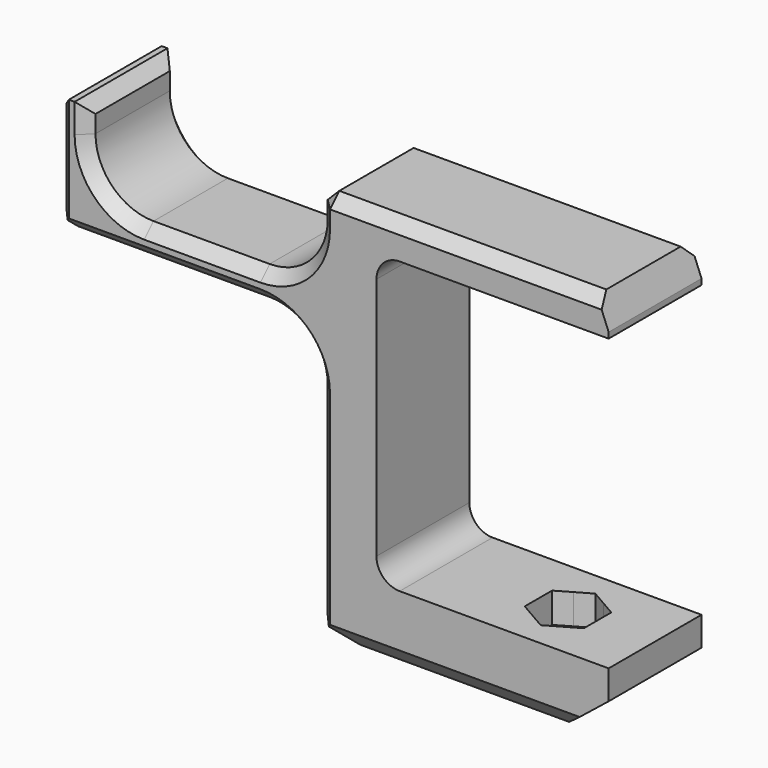
from build123d import *

# Parameters (mm, degrees)
F0_W       = 50.8
F0_H       = 6.35
F0_H_2     = 7.62
F0_H_3     = 16.51
F1_DEPTH   = 25.4
F2_R       = 12.7
F3_SIZE    = 2.54
F4_R       = 12.7
F5_SIZE    = 2.54
F6_R       = 5.08
F8_C1_SIZE = 5.08
F8_C2_SIZE = 5.08
F8_C3_SIZE = 5.08
F9_SIZE2   = 12.7
F9_SIZE    = 10.16
F10_SIZE2  = 6.35
F10_SIZE   = 2.54
F11_DEPTH  = 6.604
F12_START  = -9.906
F12_DEPTH  = 6.605
F13_D      = 8.128
F13_DEPTH  = 16.511


with BuildPart() as f1:
    # F0 (on Front) → F1 (new body)
    with BuildSketch(Plane.XZ):
        Polygon((-63.5, 19.1297054841), (-63.5, 25.4797054841), (-63.5, 44.5297054841), (-69.85, 44.5297054841), (-69.85, 19.1297054841), align=None)
        with Locations((-38.1, 22.3047054841)):
            Rectangle(F0_W, F0_H)
        Polygon((0, 36.9097054841), (0, 44.5297054841), (-12.7, 44.5297054841), (-12.7, 25.4797054841), (-12.7, 19.1297054841), (-12.7, -43.1002945159), (0, -43.1002945159), (0, -26.5902945159), align=None)
        with Locations((25.4, 40.7197054841)):
            Rectangle(F0_W, F0_H_2)
        with Locations((25.4, -34.8452945159)):
            Rectangle(F0_W, F0_H_3)
    extrude(amount=F1_DEPTH)

    # F2
    f2_edges = [f1.edges().sort_by_distance(p)[0] for p in [
        (-12.7, -12.7, 25.479705),
        (-63.5, -12.7, 25.479705),
    ]]
    fillet(f2_edges, radius=F2_R)

    # F3
    f3_edges = [f1.edges().sort_by_distance(p)[0] for p in [
        (-63.5, -12.7, 44.529705),
        (-69.85, 0, 31.829705),
        (-69.85, -12.7, 44.529705),
        (-69.85, -25.4, 31.829705),
        (-59.780256, -25.4, 29.199449),
        (-38.1, 0, 25.479705),
        (-12.7, -12.7, 44.529705),
        (19.05, -25.4, 44.529705),
        (19.05, 0, 44.529705),
        (-69.85, -12.7, 19.129705),
    ]]
    chamfer(f3_edges, length=F3_SIZE)

    # F4
    f4_edges = [f1.edges().sort_by_distance(p)[0] for p in [
        (-12.7, -12.7, 19.129705),
    ]]
    fillet(f4_edges, radius=F4_R)

    # F5
    f5_edges = [f1.edges().sort_by_distance(p)[0] for p in [
        (-12.7, -25.4, -18.335295),
        (-12.7, 0, -18.335295),
    ]]
    chamfer(f5_edges, length=F5_SIZE)

    # F6
    f6_edges = [f1.edges().sort_by_distance(p)[0] for p in [
        (0, -12.7, 36.909705),
        (0, -12.7, -26.590295),
    ]]
    fillet(f6_edges, radius=F6_R)

    # F8: chamfer of 5.08 on 5 edges, made by hand

    # F8_c1
    f8_c1_edges = [f1.edges().sort_by_distance(p)[0] for p in [
        (20.32, 0, -43.1002945159),
    ]]
    chamfer(f8_c1_edges, length=F8_C1_SIZE)

    # F8_c2
    f8_c2_edges = [f1.edges().sort_by_distance(p)[0] for p in [
        (-12.7, -13.97, -43.1002945159),
    ]]
    chamfer(f8_c2_edges, length=F8_C2_SIZE)

    # F8_c3
    f8_c3_edges = [f1.edges().sort_by_distance(p)[0] for p in [
        (21.59, -25.4, -43.1002945159),
    ]]
    chamfer(f8_c3_edges, length=F8_C3_SIZE)

    # F9
    f9_edges = [f1.edges().sort_by_distance(p)[0] for p in [
        (50.8, -12.7, -43.100295),
    ]]
    f9_side = f1.faces().sort_by_distance((50.8, -12.7, -34.415021))[0]
    chamfer(f9_edges, length=F9_SIZE, length2=F9_SIZE2, reference=f9_side)

    # F10
    f10_edges = [f1.edges().sort_by_distance(p)[0] for p in [
        (50.8, -12.7, 44.529705),
    ]]
    f10_side = f1.faces().sort_by_distance((20.32, -12.7, 44.529705))[0]
    chamfer(f10_edges, length=F10_SIZE, length2=F10_SIZE2, reference=f10_side)

    # F7 (on face) → F11 (cut)
    with BuildSketch(Plane.XY.offset(-26.5902945159)):
        with BuildLine():
            Line((25.273, -16.4394976935), (28.5114998927, -18.3092464784))
            ThreePointArc((28.5114998927, -18.3092464784), (26.1407534287, -15.9384999464), (25.273, -12.7))
            Line((25.273, -12.7), (25.273, -16.4394976935))
        make_face()
        with BuildLine():
            ThreePointArc((25.273, -12.7), (26.1407534711, -9.4614999803), (28.5115000394, -7.0907534369))
            Line((28.5115000394, -7.0907534369), (25.273, -8.9605023065))
            Line((25.273, -8.9605023065), (25.273, -12.7))
        make_face()
        with BuildLine():
            ThreePointArc((28.5115000394, -7.0907534369), (31.7500001819, -6.223), (34.9885002756, -7.0907536188))
            Line((34.9885002756, -7.0907536188), (31.75, -5.2210046129))
            Line((31.75, -5.2210046129), (28.5115000394, -7.0907534369))
        make_face()
        with BuildLine():
            ThreePointArc((34.9885002756, -7.0907536188), (37.3592466199, -9.4615001378), (38.227, -12.7))
            Line((38.227, -12.7), (38.227, -8.9605023065))
            Line((38.227, -8.9605023065), (34.9885002756, -7.0907536188))
        make_face()
        with BuildLine():
            Line((38.227, -16.4394976935), (38.227, -12.7))
            ThreePointArc((38.227, -12.7), (37.3592466025, -15.9384998923), (34.9885002155, -18.3092464159))
            Line((34.9885002155, -18.3092464159), (38.227, -16.4394976935))
        make_face()
        with BuildLine():
            Line((31.75, -20.1789953871), (34.9885002155, -18.3092464159))
            ThreePointArc((34.9885002155, -18.3092464159), (31.7500000625, -19.177), (28.5114998927, -18.3092464784))
            Line((28.5114998927, -18.3092464784), (31.75, -20.1789953871))
        make_face()
        with BuildLine():
            ThreePointArc((34.9885002155, -18.3092464159), (37.3592466025, -15.9384998923), (38.227, -12.7))
            ThreePointArc((38.227, -12.7), (37.3592466199, -9.4615001378), (34.9885002756, -7.0907536188))
            ThreePointArc((34.9885002756, -7.0907536188), (31.7500001819, -6.223), (28.5115000394, -7.0907534369))
            ThreePointArc((28.5115000394, -7.0907534369), (26.1407534711, -9.4614999803), (25.273, -12.7))
            ThreePointArc((25.273, -12.7), (26.1407534287, -15.9384999464), (28.5114998927, -18.3092464784))
            ThreePointArc((28.5114998927, -18.3092464784), (31.7500000625, -19.177), (34.9885002155, -18.3092464159))
        make_face()
    extrude(amount=-F11_DEPTH, mode=Mode.SUBTRACT)

    # F7 (on face) → F12 (cut)
    with BuildSketch(Plane.XY.offset(-26.5902945159).offset(F12_START)):
        with BuildLine():
            ThreePointArc((34.9885002155, -18.3092464159), (37.3592466025, -15.9384998923), (38.227, -12.7))
            ThreePointArc((38.227, -12.7), (37.3592466199, -9.4615001378), (34.9885002756, -7.0907536188))
            ThreePointArc((34.9885002756, -7.0907536188), (31.7500001819, -6.223), (28.5115000394, -7.0907534369))
            ThreePointArc((28.5115000394, -7.0907534369), (26.1407534711, -9.4614999803), (25.273, -12.7))
            ThreePointArc((25.273, -12.7), (26.1407534287, -15.9384999464), (28.5114998927, -18.3092464784))
            ThreePointArc((28.5114998927, -18.3092464784), (31.7500000625, -19.177), (34.9885002155, -18.3092464159))
        make_face()
        with BuildLine():
            Line((38.227, -16.4394976935), (38.227, -12.7))
            ThreePointArc((38.227, -12.7), (37.3592466025, -15.9384998923), (34.9885002155, -18.3092464159))
            Line((34.9885002155, -18.3092464159), (38.227, -16.4394976935))
        make_face()
        with BuildLine():
            ThreePointArc((28.5115000394, -7.0907534369), (31.7500001819, -6.223), (34.9885002756, -7.0907536188))
            Line((34.9885002756, -7.0907536188), (31.75, -5.2210046129))
            Line((31.75, -5.2210046129), (28.5115000394, -7.0907534369))
        make_face()
        with BuildLine():
            ThreePointArc((34.9885002756, -7.0907536188), (37.3592466199, -9.4615001378), (38.227, -12.7))
            Line((38.227, -12.7), (38.227, -8.9605023065))
            Line((38.227, -8.9605023065), (34.9885002756, -7.0907536188))
        make_face()
        with BuildLine():
            ThreePointArc((25.273, -12.7), (26.1407534711, -9.4614999803), (28.5115000394, -7.0907534369))
            Line((28.5115000394, -7.0907534369), (25.273, -8.9605023065))
            Line((25.273, -8.9605023065), (25.273, -12.7))
        make_face()
        with BuildLine():
            Line((25.273, -16.4394976935), (28.5114998927, -18.3092464784))
            ThreePointArc((28.5114998927, -18.3092464784), (26.1407534287, -15.9384999464), (25.273, -12.7))
            Line((25.273, -12.7), (25.273, -16.4394976935))
        make_face()
        with BuildLine():
            Line((31.75, -20.1789953871), (34.9885002155, -18.3092464159))
            ThreePointArc((34.9885002155, -18.3092464159), (31.7500000625, -19.177), (28.5114998927, -18.3092464784))
            Line((28.5114998927, -18.3092464784), (31.75, -20.1789953871))
        make_face()
    extrude(amount=-F12_DEPTH, mode=Mode.SUBTRACT)

    # F13 (through all, one way)
    with BuildSketch(Plane.XY.offset(-26.5902945159)):
        with Locations((31.75, -12.7)):
            Circle(F13_D / 2)
    extrude(amount=-F13_DEPTH, mode=Mode.SUBTRACT)


solid = f1.part
